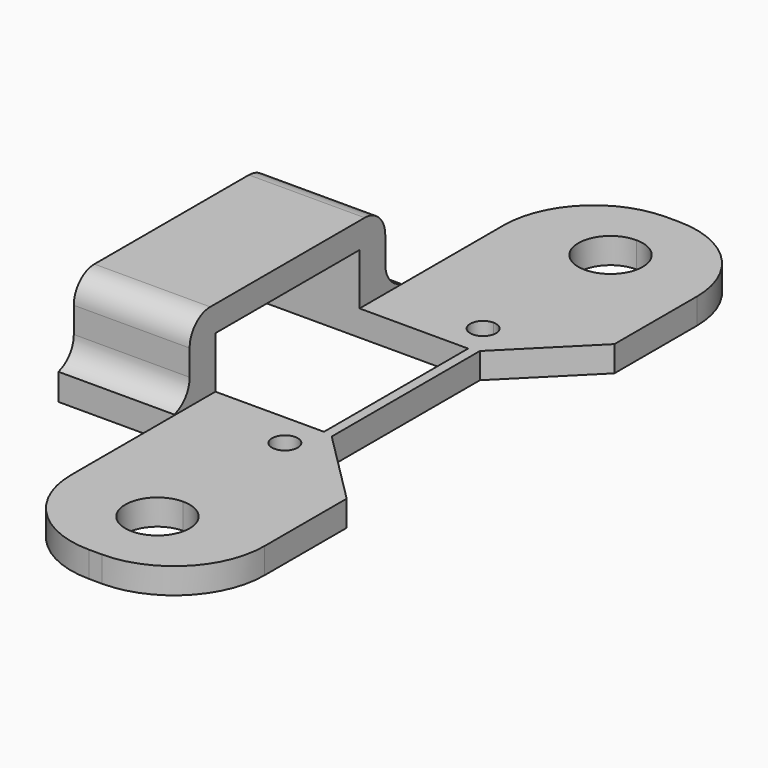
from build123d import *

# Parameters (mm, degrees)
F0_W          = 0.7558596553
F0_H          = 7
F1_DEPTH      = 2
F2_R          = 7
F4_DEPTH      = 2
F5_W          = 4
F5_H          = 2
F6_DEPTH      = 9
F8_DEPTH      = 6
F9_W          = 9
F9_H          = 2
F10_DEPTH     = 14
F11_W         = 4
F11_H         = 2
F12_DEPTH     = 9
F13_W         = 9
F13_H         = 2.5
F14_DEPTH     = 6
F15_T4_DEPTH  = 32.8601958556
F15_T9_DEPTH  = 32.8601958556
F16_T4_DEPTH  = 9
F16_T9_DEPTH  = 9
F16_T11_DEPTH = 19


# Not quite as in the source:
# - a fillet or chamfer that OpenCascade refuses, or shapes differently, is made with other operations: its cross-section is extruded or revolved along the edge and cut away or added
# - a feature names something its author has since deleted; it is built from what else it names


with BuildPart() as f1:
    # F0 (on Top) → F1 (new body)
    with BuildSketch(Plane.XY):
        Polygon((-2.7234070003, 10.5), (-7.5, 10.5), (-7.5, -10.5), (7.5, -10.5), (7.5, 10.5), (1.692557591, 10.5), (0.9366979357, 10.5), (-1.7226199852, 10.5), (-2.5201837998, 10.5), align=None)
        with Locations((1.3146277633, 14)):
            Rectangle(F0_W, F0_H)
        with Locations((1.3146277633, 21)):
            Rectangle(F0_W, F0_H)
        Polygon((-1.7226199852, 24.5), (0.9366979357, 24.5), (1.692557591, 24.5), (7.5, 24.5), (7.5, 45.5), (-7.5, 45.5), (-7.5, 24.5), (-2.7234070003, 24.5), (-2.5201837998, 24.5), align=None)
    extrude(amount=F1_DEPTH)

    # F2
    f2_edges = [f1.edges().sort_by_distance(p)[0] for p in [
        (-7.5, -10.5, 1),
        (7.5, -10.5, 1),
        (7.5, 45.5, 1),
        (-7.5, 45.5, 1),
    ]]
    fillet(f2_edges, radius=F2_R)

    # F3 (on face) → F4 (cut, through all)
    with BuildSketch(Plane.XY.offset(2)):
        with BuildLine():
            ThreePointArc((0, -7), (1.767766953, -6.267766953), (2.5, -4.5))
            ThreePointArc((2.5, -4.5), (1.767766953, -2.732233047), (0, -2))
            Line((0, -2), (0, -4.5))
            Line((0, -4.5), (0, -7))
        make_face()
        with BuildLine():
            ThreePointArc((1, 7.875), (-0.7071067812, 8.5821067812), (0, 6.875))
            ThreePointArc((0, 6.875), (0.7071067812, 7.1678932188), (1, 7.875))
        make_face()
        with BuildLine():
            Line((0, -4.5), (0, -2))
            ThreePointArc((0, -2), (-2.5, -4.5), (0, -7))
            Line((0, -7), (0, -4.5))
        make_face()
        with BuildLine():
            ThreePointArc((2.5, 39.5), (1.767766953, 41.267766953), (0, 42))
            Line((0, 42), (0, 39.5))
            Line((0, 39.5), (0, 37))
            ThreePointArc((0, 37), (1.767766953, 37.732233047), (2.5, 39.5))
        make_face()
        with BuildLine():
            ThreePointArc((1, 27.125), (0.7071067812, 27.8321067812), (0, 28.125))
            ThreePointArc((0, 28.125), (-0.7071067812, 26.4178932188), (1, 27.125))
        make_face()
        with BuildLine():
            Line((0, 39.5), (0, 42))
            ThreePointArc((0, 42), (-2.5, 39.5), (0, 37))
            Line((0, 37), (0, 39.5))
        make_face()
    extrude(amount=-F4_DEPTH, mode=Mode.SUBTRACT)

    # F5 (on face) → F6 (join)
    with BuildSketch(Plane(origin=(-7.5, 0, 0), x_dir=(0, -1, 0), z_dir=(-1, 0, 0))):
        with Locations((-8.5, 1)):
            Rectangle(F5_W, F5_H)
    extrude(amount=F6_DEPTH)

    # F7 (on face) → F8 (join)
    with BuildSketch(Plane.XY.offset(2)):
        Polygon((-8.0660292879, 10.5), (-16.5, 10.5), (-16.5, 8), (-7.5, 8), (-7.5, 10.5), align=None)
    extrude(amount=F8_DEPTH)

    # F9 (on face) → F10 (join)
    with BuildSketch(Plane(origin=(0, 10.5, 0), x_dir=(-1, 0, 0), z_dir=(0, 1, 0))):
        with Locations((12, 7)):
            Rectangle(F9_W, F9_H)
    extrude(amount=F10_DEPTH)

    # F11 (on face) → F12 (join)
    with BuildSketch(Plane(origin=(-7.5, 0, 0), x_dir=(0, -1, 0), z_dir=(-1, 0, 0))):
        with Locations((-26.5, 1)):
            Rectangle(F11_W, F11_H)
    extrude(amount=F12_DEPTH)

    # F13 (on face) → F14 (join)
    with BuildSketch(Plane.XY.offset(2)):
        with Locations((-12, 25.75)):
            Rectangle(F13_W, F13_H)
    extrude(amount=F14_DEPTH)

    # F15: chamfer of 6 on 2 edges, made by hand


with BuildPart() as f15_tool2:
    # F15_s3 → F15_t4 (new body)
    with BuildSketch(Plane.XY.offset(-15.4300979278)):
        Polygon((1.5, 10.5), (7.5, 4.5), (7.5, 10.5), align=None)
    extrude(amount=F15_T4_DEPTH)

    split(bisect_by=Plane.YZ.offset(1.692557591), keep=Keep.TOP)


with BuildPart() as f1_1:
    add(f1.part)

    # F15_t1: cut F15_tool2
    add(f15_tool2.part, mode=Mode.SUBTRACT)


with BuildPart() as f15_tool7:
    # F15_s8 → F15_t9 (new body)
    with BuildSketch(Plane.XY.offset(-15.4300979278)):
        Polygon((7.5, 30.5), (1.5, 24.5), (7.5, 24.5), align=None)
    extrude(amount=F15_T9_DEPTH)

    split(bisect_by=Plane.YZ.offset(1.692557591), keep=Keep.TOP)


with BuildPart() as f1_2:
    add(f1_1.part)

    # F15_t6: cut F15_tool7
    add(f15_tool7.part, mode=Mode.SUBTRACT)

    # F16: fillet of radius 2 on 4 edges, made by hand


with BuildPart() as f16_tool2:
    # F16_s3 → F16_t4 (new body)
    with BuildSketch(Plane.YZ.offset(-16.5)):
        with BuildLine():
            ThreePointArc((8, 4), (7.4142135624, 2.5857864376), (6, 2))
            Line((6, 2), (8, 2))
            Line((8, 2), (8, 4))
        make_face()
    extrude(amount=F16_T4_DEPTH)

    split(bisect_by=Plane.XZ.offset(-6.5), keep=Keep.BOTTOM)


with BuildPart() as f1_3:
    add(f1_2.part)

    # F16_t1: union F16_tool2
    add(f16_tool2.part)


with BuildPart() as f16_tool7:
    # F16_s8 → F16_t9 (new body)
    with BuildSketch(Plane.YZ.offset(-7.5)):
        with BuildLine():
            ThreePointArc((27, 4), (27.5857864376, 2.5857864376), (29, 2))
            Line((29, 2), (27, 2))
            Line((27, 2), (27, 4))
        make_face()
    extrude(amount=-F16_T9_DEPTH)

    split(bisect_by=Plane.XZ.offset(-28.5), keep=Keep.TOP)


with BuildPart() as f1_4:
    add(f1_3.part)

    # F16_t6: union F16_tool7
    add(f16_tool7.part)

    # F16_s12 → F16_t11 (cut)
    with BuildSketch(Plane.YZ.offset(-21.5)):
        with BuildLine():
            ThreePointArc((8, 6), (8.5857864376, 7.4142135624), (10, 8))
            Line((10, 8), (8, 8))
            Line((8, 8), (8, 6))
        make_face()
        with BuildLine():
            ThreePointArc((25, 8), (26.4142135624, 7.4142135624), (27, 6))
            Line((27, 6), (27, 8))
            Line((27, 8), (25, 8))
        make_face()
    extrude(amount=F16_T11_DEPTH, mode=Mode.SUBTRACT)


solid = f1_4.part
